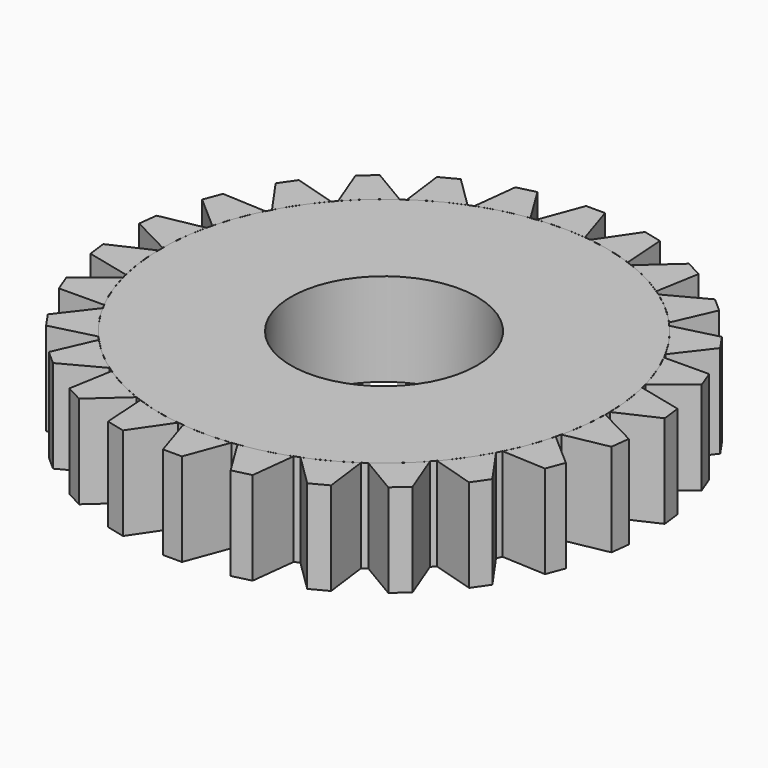
from build123d import *

# Parameters (mm, degrees)
F3_R              = 60
F4_DEPTH          = 25
F4_2_COPIES_COUNT = 26
F1_R              = 25
F5_DEPTH          = 25


# Not quite as in the source:
# - a pattern or mirror of a feature is missing from the dataset's text; its kind, count and spacing are read off the source's solid
# - a feature names something its author has since deleted; it is built from what else it names


with BuildPart() as f4:
    # F3 (on Top) → F4 (new body)
    with BuildSketch(Plane.XY):
        Circle(F3_R)
    extrude(amount=F4_DEPTH)

    # F1 (on Top) → F5 (cut)
    with BuildSketch(Plane.XY):
        Circle(F1_R)
    extrude(amount=F5_DEPTH, mode=Mode.SUBTRACT)


with BuildPart() as f4b:
    # F2 (on Top) → F4, piece 2 (new body)
    with BuildSketch(Plane.XY):
        with BuildLine():
            Line((-2.4335789598, 70.9486660947), (-6.6399739693, 59.6314576854))
            ThreePointArc((-6.6399739693, 59.6314576854), (-0.1739061559, 59.9997479715), (6.2941879381, 59.6689466825))
            Line((6.2941879381, 59.6689466825), (2.6741870575, 70.9486660947))
            Line((2.6741870575, 70.9486660947), (-2.4335789598, 70.9486660947))
        make_face()
    extrude(amount=F4_DEPTH)


with BuildPart() as f4_2_copies_1:
    # F4_2_copies: instance of F4b
    add(f4b.part.rotate(Axis((0, 0, 0), (0, 0, 1)), 1 * 360 / F4_2_COPIES_COUNT))


with BuildPart() as f4_2_copies_2:
    # F4_2_copies: instance of F4b
    add(f4b.part.rotate(Axis((0, 0, 0), (0, 0, 1)), 2 * 360 / F4_2_COPIES_COUNT))


with BuildPart() as f4_2_copies_3:
    # F4_2_copies: instance of F4b
    add(f4b.part.rotate(Axis((0, 0, 0), (0, 0, 1)), 3 * 360 / F4_2_COPIES_COUNT))


with BuildPart() as f4_2_copies_4:
    # F4_2_copies: instance of F4b
    add(f4b.part.rotate(Axis((0, 0, 0), (0, 0, 1)), 4 * 360 / F4_2_COPIES_COUNT))


with BuildPart() as f4_2_copies_5:
    # F4_2_copies: instance of F4b
    add(f4b.part.rotate(Axis((0, 0, 0), (0, 0, 1)), 5 * 360 / F4_2_COPIES_COUNT))


with BuildPart() as f4_2_copies_6:
    # F4_2_copies: instance of F4b
    add(f4b.part.rotate(Axis((0, 0, 0), (0, 0, 1)), 6 * 360 / F4_2_COPIES_COUNT))


with BuildPart() as f4_2_copies_7:
    # F4_2_copies: instance of F4b
    add(f4b.part.rotate(Axis((0, 0, 0), (0, 0, 1)), 7 * 360 / F4_2_COPIES_COUNT))


with BuildPart() as f4_2_copies_8:
    # F4_2_copies: instance of F4b
    add(f4b.part.rotate(Axis((0, 0, 0), (0, 0, 1)), 8 * 360 / F4_2_COPIES_COUNT))


with BuildPart() as f4_2_copies_9:
    # F4_2_copies: instance of F4b
    add(f4b.part.rotate(Axis((0, 0, 0), (0, 0, 1)), 9 * 360 / F4_2_COPIES_COUNT))


with BuildPart() as f4_2_copies_10:
    # F4_2_copies: instance of F4b
    add(f4b.part.rotate(Axis((0, 0, 0), (0, 0, 1)), 10 * 360 / F4_2_COPIES_COUNT))


with BuildPart() as f4_2_copies_11:
    # F4_2_copies: instance of F4b
    add(f4b.part.rotate(Axis((0, 0, 0), (0, 0, 1)), 11 * 360 / F4_2_COPIES_COUNT))


with BuildPart() as f4_2_copies_12:
    # F4_2_copies: instance of F4b
    add(f4b.part.rotate(Axis((0, 0, 0), (0, 0, 1)), 12 * 360 / F4_2_COPIES_COUNT))


with BuildPart() as f4_2_copies_13:
    # F4_2_copies: instance of F4b
    add(f4b.part.rotate(Axis((0, 0, 0), (0, 0, 1)), 13 * 360 / F4_2_COPIES_COUNT))


with BuildPart() as f4_2_copies_14:
    # F4_2_copies: instance of F4b
    add(f4b.part.rotate(Axis((0, 0, 0), (0, 0, 1)), 14 * 360 / F4_2_COPIES_COUNT))


with BuildPart() as f4_2_copies_15:
    # F4_2_copies: instance of F4b
    add(f4b.part.rotate(Axis((0, 0, 0), (0, 0, 1)), 15 * 360 / F4_2_COPIES_COUNT))


with BuildPart() as f4_2_copies_16:
    # F4_2_copies: instance of F4b
    add(f4b.part.rotate(Axis((0, 0, 0), (0, 0, 1)), 16 * 360 / F4_2_COPIES_COUNT))


with BuildPart() as f4_2_copies_17:
    # F4_2_copies: instance of F4b
    add(f4b.part.rotate(Axis((0, 0, 0), (0, 0, 1)), 17 * 360 / F4_2_COPIES_COUNT))


with BuildPart() as f4_2_copies_18:
    # F4_2_copies: instance of F4b
    add(f4b.part.rotate(Axis((0, 0, 0), (0, 0, 1)), 18 * 360 / F4_2_COPIES_COUNT))


with BuildPart() as f4_2_copies_19:
    # F4_2_copies: instance of F4b
    add(f4b.part.rotate(Axis((0, 0, 0), (0, 0, 1)), 19 * 360 / F4_2_COPIES_COUNT))


with BuildPart() as f4_2_copies_20:
    # F4_2_copies: instance of F4b
    add(f4b.part.rotate(Axis((0, 0, 0), (0, 0, 1)), 20 * 360 / F4_2_COPIES_COUNT))


with BuildPart() as f4_2_copies_21:
    # F4_2_copies: instance of F4b
    add(f4b.part.rotate(Axis((0, 0, 0), (0, 0, 1)), 21 * 360 / F4_2_COPIES_COUNT))


with BuildPart() as f4_2_copies_22:
    # F4_2_copies: instance of F4b
    add(f4b.part.rotate(Axis((0, 0, 0), (0, 0, 1)), 22 * 360 / F4_2_COPIES_COUNT))


with BuildPart() as f4_2_copies_23:
    # F4_2_copies: instance of F4b
    add(f4b.part.rotate(Axis((0, 0, 0), (0, 0, 1)), 23 * 360 / F4_2_COPIES_COUNT))


with BuildPart() as f4_2_copies_24:
    # F4_2_copies: instance of F4b
    add(f4b.part.rotate(Axis((0, 0, 0), (0, 0, 1)), 24 * 360 / F4_2_COPIES_COUNT))


with BuildPart() as f4_2_copies_25:
    # F4_2_copies: instance of F4b
    add(f4b.part.rotate(Axis((0, 0, 0), (0, 0, 1)), 25 * 360 / F4_2_COPIES_COUNT))


solid = Compound([f4.part, f4b.part, f4_2_copies_1.part, f4_2_copies_2.part, f4_2_copies_3.part, f4_2_copies_4.part, f4_2_copies_5.part, f4_2_copies_6.part, f4_2_copies_7.part, f4_2_copies_8.part, f4_2_copies_9.part, f4_2_copies_10.part, f4_2_copies_11.part, f4_2_copies_12.part, f4_2_copies_13.part, f4_2_copies_14.part, f4_2_copies_15.part, f4_2_copies_16.part, f4_2_copies_17.part, f4_2_copies_18.part, f4_2_copies_19.part, f4_2_copies_20.part, f4_2_copies_21.part, f4_2_copies_22.part, f4_2_copies_23.part, f4_2_copies_24.part, f4_2_copies_25.part])
